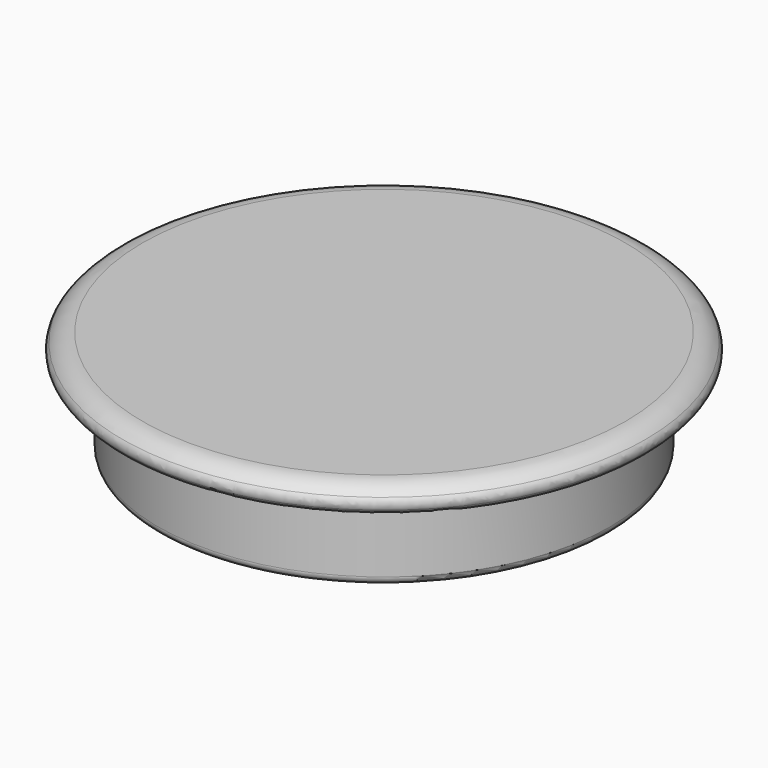
from build123d import *

# Parameters (mm, degrees)
F0_R     = 17.1
F1_DEPTH = 6
F2_R     = 20
F2_R_2   = 17.1
F3_DEPTH = 2
F4_T     = -1.2
F5_R     = 0.59999
F6_R     = 1
F8_R     = 0.7


# Not quite as in the source:
# - a fillet or chamfer that OpenCascade refuses, or shapes differently, is made with other operations: its cross-section is extruded or revolved along the edge and cut away or added
# - a fillet or chamfer is up to 0.001 mm smaller than in the source, because OpenCascade refuses the exact size


with BuildPart() as f1:
    # F0 (on Top) → F1 (new body)
    with BuildSketch(Plane.XY):
        Circle(F0_R)
    extrude(amount=F1_DEPTH)

    # F2 (on face) → F3 (join)
    with BuildSketch(Plane.XY.offset(6)):
        Circle(F2_R)
        Circle(F2_R_2, mode=Mode.SUBTRACT)
        Circle(F2_R_2)
    extrude(amount=F3_DEPTH)

    # F4
    f4_openings = [f1.faces().sort_by_distance(p)[0] for p in [
        (0, 0, 0),
    ]]
    offset(amount=F4_T, openings=f4_openings, kind=Kind.INTERSECTION)

    # F5 (radius 0.6 in the source; OpenCascade refuses exactly that, so slightly less here)
    f5_edges = [f1.edges().sort_by_distance(p)[0] for p in [
        (-15.9, 0, 0),
        (-17.1, 0, 0),
    ]]
    fillet(f5_edges, radius=F5_R)

    # F6
    f6_edges = [f1.edges().sort_by_distance(p)[0] for p in [
        (-17.1, 0, 6),
        (-20, 0, 6),
        (-15.9, 0, 6.8),
    ]]
    fillet(f6_edges, radius=F6_R)

    # F7: fillet of radius 2 on 1 edges, made by hand

    # F7_s1 → F7_t2 (revolve, cut)
    with BuildSketch(Plane.XZ):
        with BuildLine():
            ThreePointArc((20, 7), (19.2679491924, 7.7320508076), (18.2679491924, 8))
            Line((18.2679491924, 8), (18.2679491924, 8.04))
            Line((18.2679491924, 8.04), (20, 8.04))
            Line((20, 8.04), (20.04, 8))
            ThreePointArc((20.04, 8), (20.04, 7.5), (20.0346410162, 7.02))
            Line((20.0346410162, 7.02), (20, 7))
        make_face()
    revolve(axis=Axis((0, 0, 8), (0, 0, 1)), mode=Mode.SUBTRACT)

    # F8
    f8_edges = [f1.edges().sort_by_distance(p)[0] for p in [
        (-20, 0, 7),
    ]]
    fillet(f8_edges, radius=F8_R)


solid = f1.part
